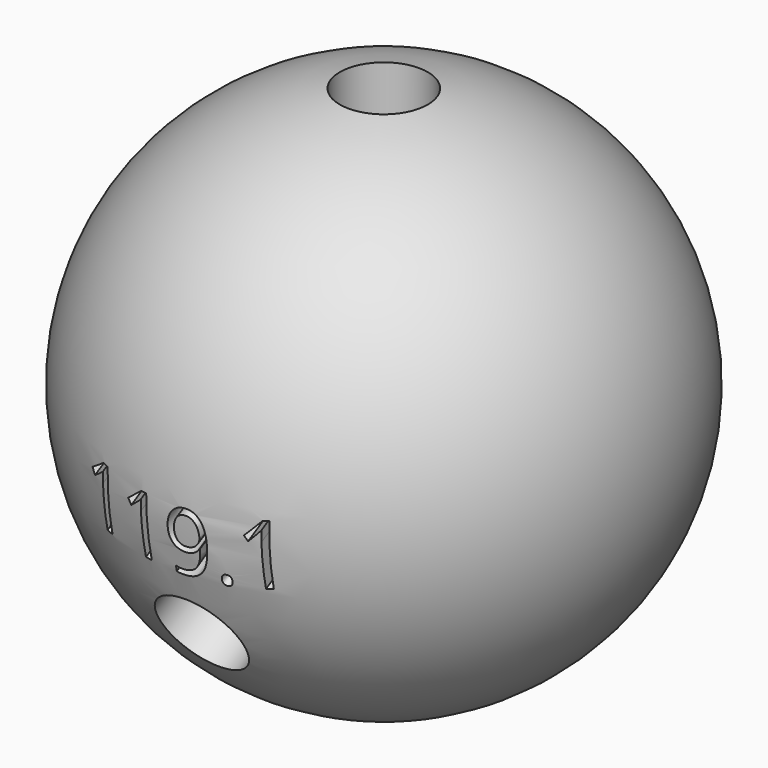
from build123d import *

# Parameters (mm, degrees)
F5_R          = 3.175
F6_DEPTH      = 76.2
F7_ANGLE      = 119.1
F8_ANGLE      = 121.5
F10_TEXT_SIZE = 5.7784387738
F11_DEPTH     = 6.35
F13_TEXT_SIZE = 6.645384969
F14_DEPTH     = 7.62


# Not quite as in the source:
# - Text() gives the source's letters only with a copy of the font that has no kerning and outlines rounded to 1/6400 em; it was checked with that copy


with BuildPart() as f2:
    # F0 (on Front) → F2 (revolve)
    with BuildSketch(Plane.XZ):
        with BuildLine():
            Line((0, -19.05), (0, 19.05))
            ThreePointArc((0, 19.05), (-19.05, 0), (0, -19.05))
        make_face()
    revolve(axis=Axis((0, 0, 0), (0, 0, 1)))

    # F10 (on offset) → F11 (cut)
    with BuildSketch(Plane(origin=(0, -17.7550515721, -9.8823349302), x_dir=(1, 0, 0), z_dir=(0, -0.873772223, -0.4863353804))):
        with Locations((-7.3158596642, 5.1700836048)):
            Text('119.1', F10_TEXT_SIZE, font='Open Sans', text_align=(TextAlign.LEFT, TextAlign.BOTTOM))
    extrude(amount=-F11_DEPTH, mode=Mode.SUBTRACT)

    # F13 (on offset) → F14 (cut)
    with BuildSketch(Plane(origin=(0, 17.703064642, -9.9751642735), x_dir=(-1, 0, 0), z_dir=(0, 0.8712138111, -0.4909037536))):
        with Locations((-8.5071311017, 6.5399650484)):
            Text('121.5', F13_TEXT_SIZE, font='Open Sans', text_align=(TextAlign.LEFT, TextAlign.BOTTOM))
    extrude(amount=-F14_DEPTH, mode=Mode.SUBTRACT)


with BuildPart() as f6:
    # F5 (on offset) → F6 (new body)
    with BuildSketch(Plane.XY.offset(7.62)):
        Circle(F5_R)
    extrude(amount=F6_DEPTH)


with BuildPart() as f7_1:
    # F7: copy of F6
    add(f6.part.rotate(Axis((38.1614528596, 0, 0), (1, 0, 0)), F7_ANGLE))


with BuildPart() as f8_1:
    # F8: copy of F7_1
    add(f7_1.part.rotate(Axis((38.1614528596, 0, 0), (1, 0, 0)), F8_ANGLE))


with BuildPart() as f2_1:
    add(f2.part)

    # F15: cut F6, F7_1, F8_1
    add(f6.part, mode=Mode.SUBTRACT)
    add(f7_1.part, mode=Mode.SUBTRACT)
    add(f8_1.part, mode=Mode.SUBTRACT)


solid = f2_1.part
